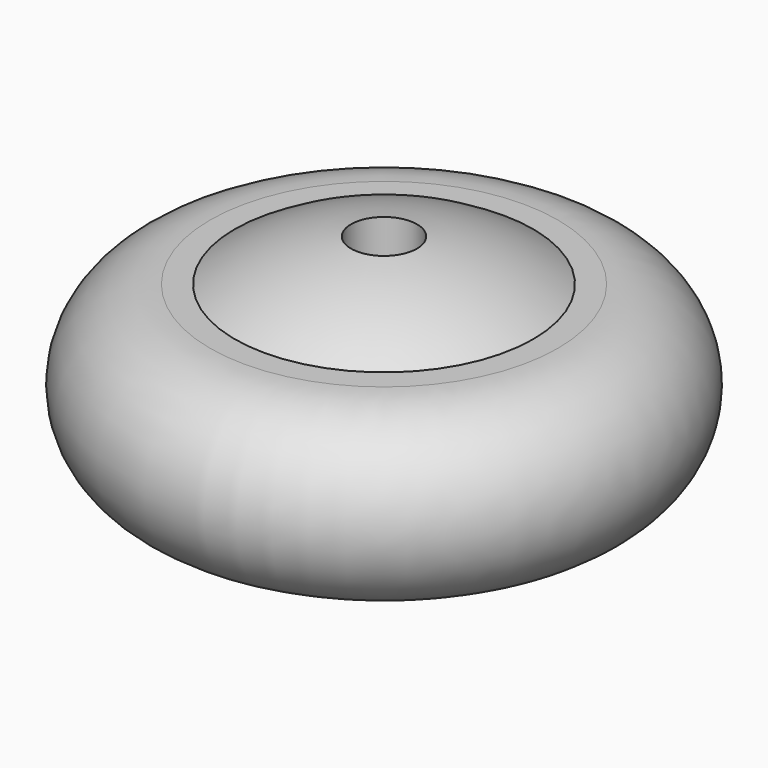
from build123d import *

# Parameters (mm, degrees)
F2_R          = 1.5
F3_DEPTH      = 5.995994212
F3_DEPTH_BACK = 6.0002622918


with BuildPart() as f1:
    # F0 (on Front) → F1 (revolve)
    with BuildSketch(Plane.XZ):
        with BuildLine():
            Line((-7.756281148, -3.9925682363), (-6.7856144907, -3.9928719014))
            ThreePointArc((-6.7856144907, -3.9928719014), (-3.5374092838, -5.4840198421), (0, -5.994994212))
            Line((0, -5.994994212), (0, 5.9992622918))
            ThreePointArc((0, 5.9992622918), (-3.5358103027, 5.4887595917), (-6.7828140924, 3.9989495724))
            Line((-6.7828140924, 3.9989495724), (-7.9061036088, 3.9988977816))
            ThreePointArc((-7.9061036088, 3.9988977816), (-11.9963821429, 0.1700875292), (-8.2462168891, -3.9924149638))
            Line((-8.2462168891, -3.9924149638), (-7.756281148, -3.9925682363))
        make_face()
        with BuildLine():
            ThreePointArc((-8.2462168891, -3.9924149638), (-8.0012513674, -3.9999998043), (-7.756281148, -3.9925682363))
            Line((-7.756281148, -3.9925682363), (-8.2462168891, -3.9924149638))
        make_face()
    revolve(axis=Axis((0, 0, 0.0021340399), (0, 0, -1)))

    # F2 (on Top) → F3 (cut, two sides)
    with BuildSketch(Plane.XY) as f3_sk:
        Circle(F2_R)
    extrude(amount=-F3_DEPTH, mode=Mode.SUBTRACT)
    extrude(f3_sk.sketch, amount=F3_DEPTH_BACK, mode=Mode.SUBTRACT)


solid = f1.part
